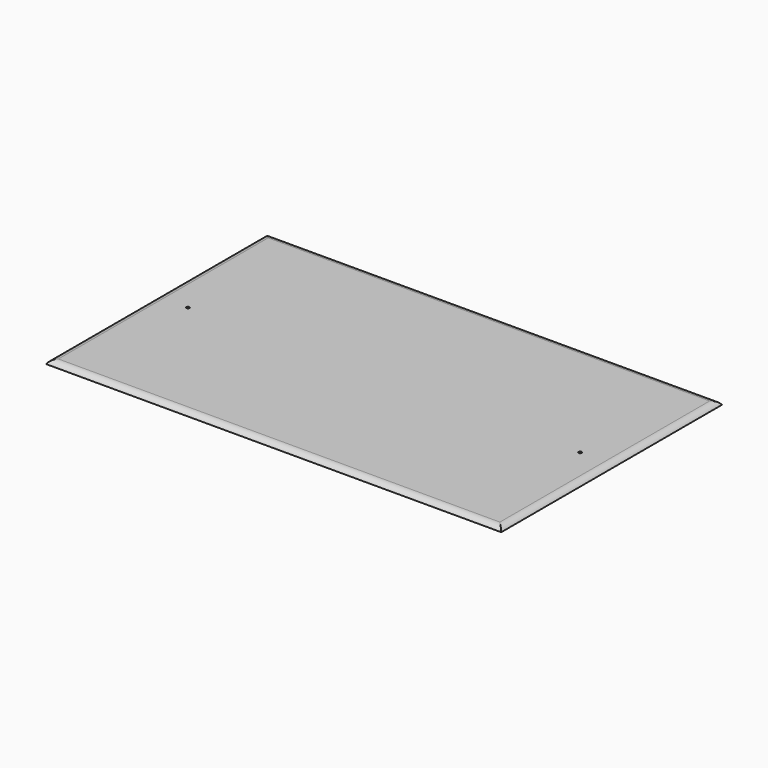
from build123d import *

# Parameters (mm, degrees)
F0_W        = 1416.05
F0_H        = 838.2
F0_R        = 4.7625
F1_DEPTH    = 12.7
F2_T1_DEPTH = 1576.8352262806
F2_T3_DEPTH = 998.9852262806


# Not quite as in the source:
# - a fillet or chamfer that OpenCascade refuses, or shapes differently, is made with other operations: its cross-section is extruded or revolved along the edge and cut away or added
# - a feature names something its author has since deleted; it is built from what else it names


with BuildPart() as f1:
    # F0 (on Top) → F1 (new body)
    with BuildSketch(Plane.XY):
        Polygon((-101.6, 812.8255558279), (-101.6, -76.1744441721), (1365.25, -76.1744441721), (1365.25, 736.6255558279), (1365.25, 812.8255558279), align=None)
        with Locations((631.825, 368.3255558279)):
            Rectangle(F0_W, F0_H, mode=Mode.SUBTRACT)
        with Locations((631.825, 368.3255558279)):
            Rectangle(F0_W, F0_H)
        with Locations((0, 368.3255558279)):
            Circle(F0_R, mode=Mode.SUBTRACT)
        with Locations((1263.65, 368.3255558279)):
            Circle(F0_R, mode=Mode.SUBTRACT)
    extrude(amount=F1_DEPTH)

    # F2: fillet of radius 25.4 on 4 edges, made by hand

    # F2_s2 → F2_t1 (cut)
    with BuildSketch(Plane.YZ.offset(-156.5926131403)):
        with BuildLine():
            ThreePointArc((-76.1744441721, 0), (-66.8773989159, 9.2970452561), (-54.1773989159, 12.7))
            Line((-54.1773989159, 12.7), (-76.1744441721, 12.7))
            Line((-76.1744441721, 12.7), (-76.1744441721, 0))
        make_face()
        with BuildLine():
            ThreePointArc((812.8255558279, 0), (803.5285105718, 9.2970452561), (790.8285105718, 12.7))
            Line((790.8285105718, 12.7), (812.8255558279, 12.7))
            Line((812.8255558279, 12.7), (812.8255558279, 0))
        make_face()
    extrude(amount=F2_T1_DEPTH, mode=Mode.SUBTRACT)

    # F2_s4 → F2_t3 (cut)
    with BuildSketch(Plane.XZ.offset(-867.8181689683)):
        with BuildLine():
            ThreePointArc((-101.6, 0), (-92.3029547439, 9.2970452561), (-79.6029547439, 12.7))
            Line((-79.6029547439, 12.7), (-101.6, 12.7))
            Line((-101.6, 12.7), (-101.6, 0))
        make_face()
        with BuildLine():
            ThreePointArc((1365.25, 0), (1355.9529547439, 9.2970452561), (1343.2529547439, 12.7))
            Line((1343.2529547439, 12.7), (1365.25, 12.7))
            Line((1365.25, 12.7), (1365.25, 0))
        make_face()
    extrude(amount=F2_T3_DEPTH, mode=Mode.SUBTRACT)


solid = f1.part
